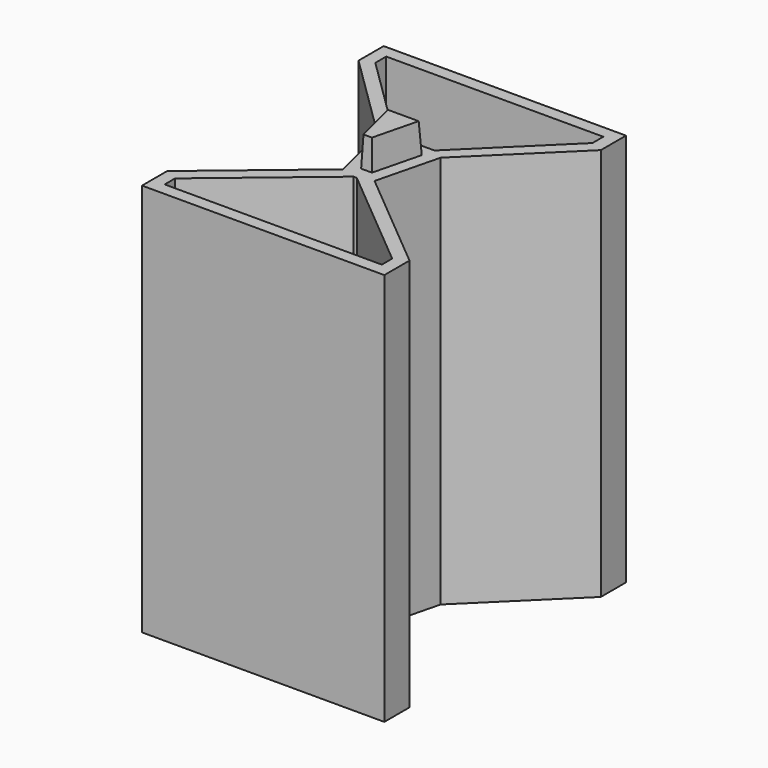
from build123d import *

# Parameters (mm, degrees)
F1_DEPTH     = 125
F2_DEPTH     = 10
F4_DEPTH     = 9.5
F5_T4_DEPTH  = 67.5870629671
F5_T9_DEPTH  = 55.4775446264
F5_T14_DEPTH = 67.5870629671
F5_T19_DEPTH = 63.0395446265


# Not quite as in the source:
# - a fillet or chamfer that OpenCascade refuses, or shapes differently, is made with other operations: its cross-section is extruded or revolved along the edge and cut away or added
# - a feature names something its author has since deleted; it is built from what else it names


with BuildPart() as f1:
    # F0 (on Top) → F1 (new body)
    with BuildSketch(Plane.XY):
        Polygon((-38.5, -38), (-38.5, -48), (38.5, -48), (38.5, -38), (5, -10), (10, 10), (38.5000000008, 38), (38.5, 48), (-38.5, 48), (-38.5000000011, 38), (-10, 10), (-5, -10), align=None)
        Polygon((-0.5119467155, -11.462), (0.5119467155, -11.462), (34.5, -39.8699251333), (34.5, -44), (-34.5, -44), (-34.5, -39.8699251333), align=None, mode=Mode.SUBTRACT)
        Polygon((-5.5209720151, 8.1640000003), (5.5209720151, 8.1640000003), (1.739972015, -6.96), (-1.739972015, -6.96), align=None, mode=Mode.SUBTRACT)
        Polygon((34.5000000007, 39.6776277195), (6.3932717857, 12.0640000003), (-6.3932717857, 12.0640000003), (-34.5000000007, 39.6776277195), (-34.5000000005, 44), (34.5000000003, 44), align=None, mode=Mode.SUBTRACT)
        Polygon((1.739972015, -6.96), (5.5209720151, 8.1640000003), (-5.5209720151, 8.1640000003), (-1.739972015, -6.96), align=None)
    extrude(amount=F1_DEPTH)

    # F0 (on Top) → F2 (cut)
    with BuildSketch(Plane.XY):
        Polygon((1.739972015, -6.96), (5.5209720151, 8.1640000003), (-5.5209720151, 8.1640000003), (-1.739972015, -6.96), align=None)
    extrude(amount=F2_DEPTH, mode=Mode.SUBTRACT)

    # F3 (on face) → F4 (join)
    with BuildSketch(Plane.XY.offset(125)):
        Polygon((1.739972015, -6.96), (5.5209720151, 8.1640000003), (-5.5209720151, 8.1640000003), (-1.739972015, -6.96), align=None)
    extrude(amount=F4_DEPTH)

    # F5: chamfer of 10 x 0.5 on 4 edges, made by hand


with BuildPart() as f5_tool2:
    # F5_s3 → F5_t4 (new body)
    with BuildSketch(Plane(origin=(-7.8409310443, -31.3637241773, 0), x_dir=(0, 0, 1), z_dir=(0.242535625, 0.9701425001, 0))):
        Polygon((124.5, 3.3760687511), (134.5, 2.8760687511), (134.5, 3.3760687511), align=None)
    extrude(amount=F5_T4_DEPTH)

    split(bisect_by=Plane.XY.offset(125), keep=Keep.TOP)


with BuildPart() as f1_1:
    add(f1.part)

    # F5_t1: cut F5_tool2
    add(f5_tool2.part, mode=Mode.SUBTRACT)


with BuildPart() as f5_tool7:
    # F5_s8 → F5_t9 (new body)
    with BuildSketch(Plane.YZ.offset(-27.7387723132)):
        Polygon((-6.96, 124.5), (-6.46, 134.5), (-6.96, 134.5), align=None)
    extrude(amount=F5_T9_DEPTH)

    split(bisect_by=Plane.XY.offset(125), keep=Keep.TOP)


with BuildPart() as f1_2:
    add(f1_1.part)

    # F5_t6: cut F5_tool7
    add(f5_tool7.part, mode=Mode.SUBTRACT)


with BuildPart() as f5_tool12:
    # F5_s13 → F5_t14 (new body)
    with BuildSketch(Plane(origin=(-8.5513395168, 34.2053580671, 0), x_dir=(0, 0, 1), z_dir=(0.242535625, -0.9701425001, 0))):
        Polygon((124.5, 3.3760687511), (134.5, 2.8760687511), (134.5, 3.3760687511), align=None)
    extrude(amount=F5_T14_DEPTH)

    split(bisect_by=Plane.XY.offset(125), keep=Keep.TOP)


with BuildPart() as f1_3:
    add(f1_2.part)

    # F5_t11: cut F5_tool12
    add(f5_tool12.part, mode=Mode.SUBTRACT)


with BuildPart() as f5_tool17:
    # F5_s18 → F5_t19 (new body)
    with BuildSketch(Plane.YZ.offset(31.5197723133)):
        Polygon((8.1640000003, 124.5), (7.6640000003, 134.5), (8.1640000003, 134.5), align=None)
    extrude(amount=-F5_T19_DEPTH)

    split(bisect_by=Plane.XY.offset(125), keep=Keep.TOP)


with BuildPart() as f1_4:
    add(f1_3.part)

    # F5_t16: cut F5_tool17
    add(f5_tool17.part, mode=Mode.SUBTRACT)


solid = f1_4.part
